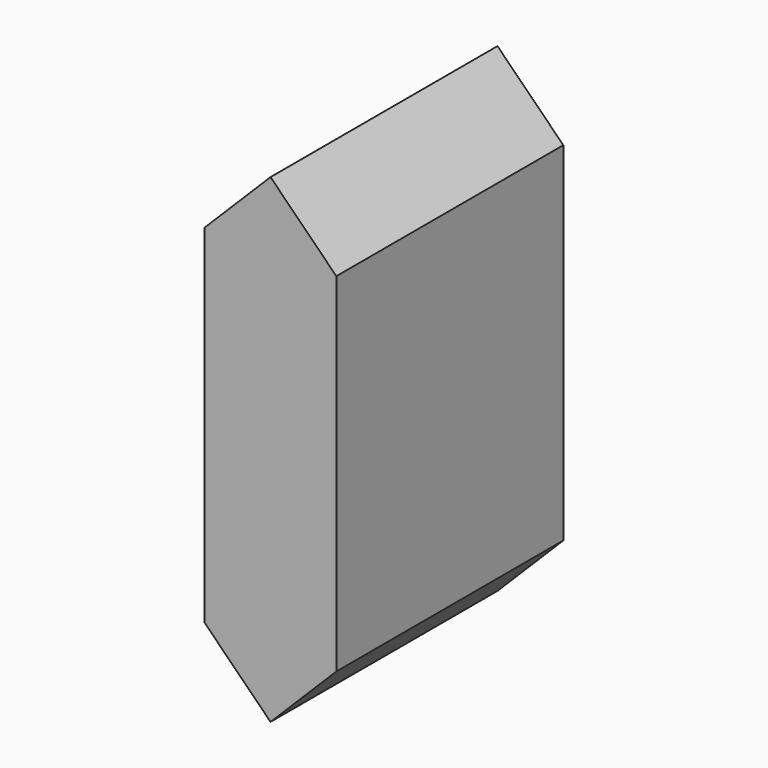
from build123d import *

# Parameters (mm, degrees)
F1_DEPTH = 0.6
F2_DEPTH = 25
F3_W     = 0.8
F3_H     = 40
F7_DEPTH = 2


with BuildPart() as f1:
    # F0 (on Front) → F1 (new body)
    with BuildSketch(Plane.XZ):
        Polygon((0, -20), (0, 20), (-5, 15), (-5, -15), align=None)
        Polygon((-5, 15), (0, 20), (0, 21.1313708499), (-5.8, 15.3313708499), (-5.8, -15.3313708499), (0, -21.1313708499), (0, -20), (-5, -15), align=None)
    extrude(amount=-F1_DEPTH)

    # F0 (on Front) → F2 (join)
    with BuildSketch(Plane.XZ):
        Polygon((-5, 15), (0, 20), (0, 21.1313708499), (-5.8, 15.3313708499), (-5.8, -15.3313708499), (0, -21.1313708499), (0, -20), (-5, -15), align=None)
    extrude(amount=-F2_DEPTH)

    # F3 (on face) → F4 (join, up to the next surface of F1)
    with BuildSketch(Plane.YZ):
        with Locations((24.6, 0)):
            Rectangle(F3_W, F3_H)
        with BuildLine():
            ThreePointArc((8.2, -20), (16.4, 0), (8.2, 20))
            Line((8.2, 20), (7.6, 20))
            ThreePointArc((7.6, 20), (15.8, 0), (7.6, -20))
            Line((7.6, -20), (8.2, -20))
        make_face()
    extrude(until=Until.NEXT, dir=(-1, 0, 0))

    # F5: F1 across face


with BuildPart() as f1_1:
    add(f1.part)
    add(f1.part.mirror(Plane(origin=(0, 13.3750956502, 0), x_dir=(0, 1, 0), z_dir=(1, 0, 0))))

    # F6 (on face) → F7 (cut)
    with BuildSketch(Plane(origin=(0, 25, 0), x_dir=(-1, 0, 0), z_dir=(0, 1, 0))):
        with BuildLine():
            ThreePointArc((2.65, 8.5), (-1.8738329701, 10.3738329701), (0, 5.85))
            ThreePointArc((0, 5.85), (1.8738329701, 6.6261670299), (2.65, 8.5))
        make_face()
        with BuildLine():
            ThreePointArc((2.65, -8.5), (1.8738329701, -6.6261670299), (0, -5.85))
            ThreePointArc((0, -5.85), (-1.8738329701, -10.3738329701), (2.65, -8.5))
        make_face()
    extrude(amount=-F7_DEPTH, mode=Mode.SUBTRACT)


solid = f1_1.part
